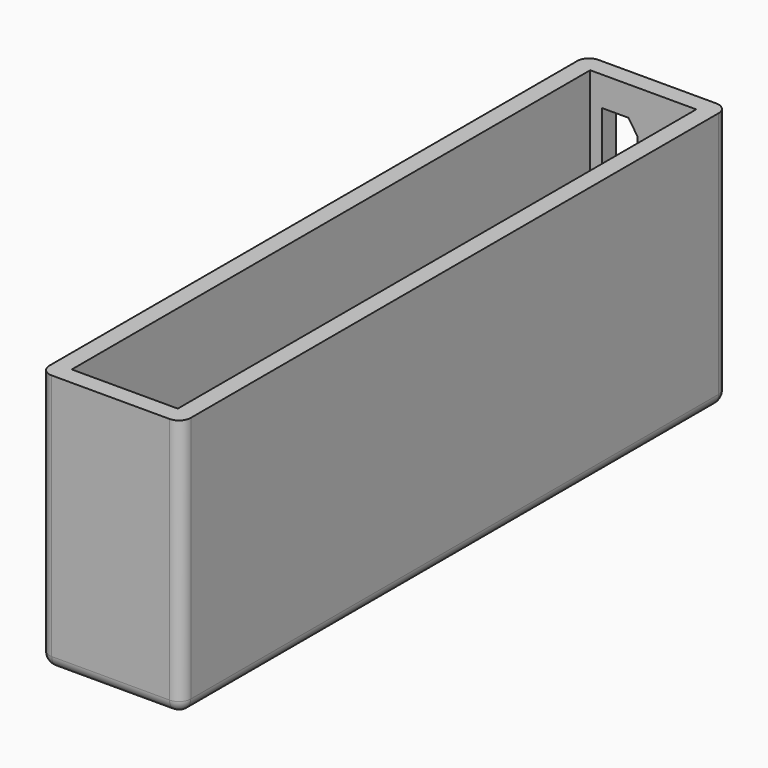
from build123d import *

# Parameters (mm, degrees)
F0_W          = 24
F0_H          = 116
F1_DEPTH      = 44
F2_T          = -3
F3_W          = 8.5
F3_H          = 16.5
F3_W_2        = 10.6
F3_H_2        = 12.5
F4_DEPTH      = 25
F5_W          = 6
F5_H          = 15.5
F6_DEPTH      = 25
F7_SIZE2      = 2.25
F7_SIZE       = 1.5
F9_DEPTH      = 7
F10_R         = 2.4
F11_DEPTH     = 1.6
F12_R         = 2
F13_T1_DEPTH  = 47
F13_S5_W      = 2
F13_S5_H      = 2
F13_T6_DEPTH  = 2
F13_S11_W     = 2
F13_S11_H     = 2
F13_T12_DEPTH = 2
F13_S17_W     = 2
F13_S17_H     = 2
F13_T18_DEPTH = 2
F13_S23_W     = 2
F13_S23_H     = 2
F13_T24_DEPTH = 2


# Not quite as in the source:
# - a fillet or chamfer that OpenCascade refuses, or shapes differently, is made with other operations: its cross-section is extruded or revolved along the edge and cut away or added


with BuildPart() as f1:
    # F0 (on Top) → F1 (new body)
    with BuildSketch(Plane.XY):
        Rectangle(F0_W, F0_H)
    extrude(amount=F1_DEPTH)

    # F2
    f2_openings = [f1.faces().sort_by_distance(p)[0] for p in [
        (0, 0, 44),
    ]]
    offset(amount=F2_T, openings=f2_openings)

    # F3 (on face) → F4 (cut)
    with BuildSketch(Plane(origin=(0, 0, 0), x_dir=(1, 0, 0), z_dir=(0, 0, -1))):
        with Locations((-4.75, 9.75)):
            Rectangle(F3_W, F3_H)
        with Locations((-3.7, -11.75)):
            Rectangle(F3_W_2, F3_H_2)
    extrude(amount=-F4_DEPTH, mode=Mode.SUBTRACT)

    # F5 (on face) → F6 (cut)
    with BuildSketch(Plane(origin=(0, 58, 0), x_dir=(-1, 0, 0), z_dir=(0, 1, 0))):
        with Locations((4, 31.25)):
            Rectangle(F5_W, F5_H)
    extrude(amount=-F6_DEPTH, mode=Mode.SUBTRACT)

    # F7
    f7_edges = [f1.edges().sort_by_distance(p)[0] for p in [
        (-1, 56.5, 23.5),
        (-1, 56.5, 39),
    ]]
    chamfer(f7_edges, length=F7_SIZE, length2=F7_SIZE2)

    # F8 (on face) → F9 (join)
    with BuildSketch(Plane.XY.offset(3)):
        Polygon((4.6, 21), (-9, 21), (-9, 18), (1.6, 18), (1.6, 5.5), (-9, 5.5), (-9, 2.5), (4.6, 2.5), align=None)
        Polygon((-9, -18), (-9, -21), (2.5, -21), (2.5, 1.5), (-9, 1.5), (-9, -1.5), (-0.5, -1.5), (-0.5, -18), align=None)
    extrude(amount=F9_DEPTH)

    # F10 (on face) → F11 (join)
    with BuildSketch(Plane(origin=(-12, 0, 0), x_dir=(0, -1, 0), z_dir=(-1, 0, 0))):
        with Locations((-52, 6)):
            Circle(F10_R)
        with Locations((-52, 14)):
            Circle(F10_R)
        with Locations((-52, 22)):
            Circle(F10_R)
        with Locations((-52, 30)):
            Circle(F10_R)
        with Locations((-52, 38)):
            Circle(F10_R)
        with Locations((-44, 6)):
            Circle(F10_R)
        with Locations((-44, 14)):
            Circle(F10_R)
        with Locations((-44, 22)):
            Circle(F10_R)
        with Locations((-44, 30)):
            Circle(F10_R)
        with Locations((-44, 38)):
            Circle(F10_R)
        with Locations((-36, 6)):
            Circle(F10_R)
        with Locations((-36, 14)):
            Circle(F10_R)
        with Locations((-36, 22)):
            Circle(F10_R)
        with Locations((-36, 30)):
            Circle(F10_R)
        with Locations((-36, 38)):
            Circle(F10_R)
        with Locations((-28, 6)):
            Circle(F10_R)
        with Locations((-28, 14)):
            Circle(F10_R)
        with Locations((-28, 22)):
            Circle(F10_R)
        with Locations((-28, 30)):
            Circle(F10_R)
        with Locations((-28, 38)):
            Circle(F10_R)
        with Locations((-20, 6)):
            Circle(F10_R)
        with Locations((-20, 14)):
            Circle(F10_R)
        with Locations((-20, 22)):
            Circle(F10_R)
        with Locations((-20, 30)):
            Circle(F10_R)
        with Locations((-20, 38)):
            Circle(F10_R)
        with Locations((-12, 6)):
            Circle(F10_R)
        with Locations((-12, 14)):
            Circle(F10_R)
        with Locations((-12, 22)):
            Circle(F10_R)
        with Locations((-12, 30)):
            Circle(F10_R)
        with Locations((-12, 38)):
            Circle(F10_R)
        with Locations((-4, 6)):
            Circle(F10_R)
        with Locations((-4, 14)):
            Circle(F10_R)
        with Locations((-4, 22)):
            Circle(F10_R)
        with Locations((-4, 30)):
            Circle(F10_R)
        with Locations((-4, 38)):
            Circle(F10_R)
        with Locations((4, 6)):
            Circle(F10_R)
        with Locations((4, 14)):
            Circle(F10_R)
        with Locations((4, 22)):
            Circle(F10_R)
        with Locations((4, 30)):
            Circle(F10_R)
        with Locations((4, 38)):
            Circle(F10_R)
        with Locations((12, 6)):
            Circle(F10_R)
        with Locations((12, 14)):
            Circle(F10_R)
        with Locations((12, 22)):
            Circle(F10_R)
        with Locations((12, 30)):
            Circle(F10_R)
        with Locations((12, 38)):
            Circle(F10_R)
        with Locations((20, 6)):
            Circle(F10_R)
        with Locations((20, 14)):
            Circle(F10_R)
        with Locations((20, 22)):
            Circle(F10_R)
        with Locations((20, 30)):
            Circle(F10_R)
        with Locations((20, 38)):
            Circle(F10_R)
        with Locations((28, 6)):
            Circle(F10_R)
        with Locations((28, 14)):
            Circle(F10_R)
        with Locations((28, 22)):
            Circle(F10_R)
        with Locations((28, 30)):
            Circle(F10_R)
        with Locations((28, 38)):
            Circle(F10_R)
        with Locations((36, 6)):
            Circle(F10_R)
        with Locations((36, 14)):
            Circle(F10_R)
        with Locations((36, 22)):
            Circle(F10_R)
        with Locations((36, 30)):
            Circle(F10_R)
        with Locations((36, 38)):
            Circle(F10_R)
        with Locations((44, 6)):
            Circle(F10_R)
        with Locations((44, 14)):
            Circle(F10_R)
        with Locations((44, 22)):
            Circle(F10_R)
        with Locations((44, 30)):
            Circle(F10_R)
        with Locations((44, 38)):
            Circle(F10_R)
        with Locations((52, 6)):
            Circle(F10_R)
        with Locations((52, 14)):
            Circle(F10_R)
        with Locations((52, 22)):
            Circle(F10_R)
        with Locations((52, 30)):
            Circle(F10_R)
        with Locations((52, 38)):
            Circle(F10_R)
    extrude(amount=F11_DEPTH)

    # F12
    f12_edges = [f1.edges().sort_by_distance(p)[0] for p in [
        (12, 0, 0),
        (0, -58, 0),
        (-12, 0, 0),
        (0, 58, 0),
    ]]
    fillet(f12_edges, radius=F12_R)

    # F13: fillet of radius 2 on 4 edges, made by hand

    # F13_s2 → F13_t1 (cut)
    with BuildSketch(Plane.XY.offset(2)):
        with BuildLine():
            ThreePointArc((-12, -56), (-11.4142135624, -57.4142135624), (-10, -58))
            Line((-10, -58), (-12, -58))
            Line((-12, -58), (-12, -56))
        make_face()
        with BuildLine():
            ThreePointArc((12, -56), (11.4142135624, -57.4142135624), (10, -58))
            Line((10, -58), (12, -58))
            Line((12, -58), (12, -56))
        make_face()
        with BuildLine():
            ThreePointArc((10, 58), (11.4142135624, 57.4142135624), (12, 56))
            Line((12, 56), (12, 58))
            Line((12, 58), (10, 58))
        make_face()
        with BuildLine():
            ThreePointArc((-10, 58), (-11.4142135624, 57.4142135624), (-12, 56))
            Line((-12, 56), (-12, 58))
            Line((-12, 58), (-10, 58))
        make_face()
    extrude(amount=F13_T1_DEPTH, mode=Mode.SUBTRACT)


with BuildPart() as f13_tool4:
    # F13_s5 → F13_t6 (new body)
    with BuildSketch(Plane.XZ.offset(-56)):
        with Locations((-11, 1)):
            Rectangle(F13_S5_W, F13_S5_H)
    extrude(amount=-F13_T6_DEPTH)

    # F13_s7 → F13_t8 (revolve, cut)
    with BuildSketch(Plane(origin=(-10, 56, 2), x_dir=(0.7071067812, 0, 0.7071067812), z_dir=(-0.7071067812, 0, 0.7071067812))):
        with BuildLine():
            ThreePointArc((0, -2), (2, 0), (0, 2))
            Line((0, 2), (0, -2))
        make_face()
    revolve(axis=Axis((-10, 56, 2), (0, 1, 0)), mode=Mode.SUBTRACT)


with BuildPart() as f1_1:
    add(f1.part)

    # F13_t3: cut F13_tool4
    add(f13_tool4.part, mode=Mode.SUBTRACT)


with BuildPart() as f13_tool10:
    # F13_s11 → F13_t12 (new body)
    with BuildSketch(Plane.XZ.offset(-56)):
        with Locations((11, 1)):
            Rectangle(F13_S11_W, F13_S11_H)
    extrude(amount=-F13_T12_DEPTH)

    # F13_s13 → F13_t14 (revolve, cut)
    with BuildSketch(Plane(origin=(10, 56, 2), x_dir=(-0.7071067812, 0, 0.7071067812), z_dir=(-0.7071067812, 0, -0.7071067812))):
        with BuildLine():
            ThreePointArc((0, -2), (2, 0), (0, 2))
            Line((0, 2), (0, -2))
        make_face()
    revolve(axis=Axis((10, 56, 2), (0, 1, 0)), mode=Mode.SUBTRACT)


with BuildPart() as f1_2:
    add(f1_1.part)

    # F13_t9: cut F13_tool10
    add(f13_tool10.part, mode=Mode.SUBTRACT)


with BuildPart() as f13_tool16:
    # F13_s17 → F13_t18 (new body)
    with BuildSketch(Plane.YZ.offset(10)):
        with Locations((-57, 1)):
            Rectangle(F13_S17_W, F13_S17_H)
    extrude(amount=F13_T18_DEPTH)

    # F13_s19 → F13_t20 (revolve, cut)
    with BuildSketch(Plane(origin=(10, -56, 2), x_dir=(0, 0.7071067812, 0.7071067812), z_dir=(0, 0.7071067812, -0.7071067812))):
        with BuildLine():
            ThreePointArc((0, -2), (2, 0), (0, 2))
            Line((0, 2), (0, -2))
        make_face()
    revolve(axis=Axis((10, -56, 2), (1, 0, 0)), mode=Mode.SUBTRACT)


with BuildPart() as f1_3:
    add(f1_2.part)

    # F13_t15: cut F13_tool16
    add(f13_tool16.part, mode=Mode.SUBTRACT)


with BuildPart() as f13_tool22:
    # F13_s23 → F13_t24 (new body)
    with BuildSketch(Plane.YZ.offset(-10)):
        with Locations((-57, 1)):
            Rectangle(F13_S23_W, F13_S23_H)
    extrude(amount=-F13_T24_DEPTH)

    # F13_s25 → F13_t26 (revolve, cut)
    with BuildSketch(Plane(origin=(-10, -56, 2), x_dir=(0, 0.7071067812, 0.7071067812), z_dir=(0, -0.7071067812, 0.7071067812))):
        with BuildLine():
            ThreePointArc((0, -2), (2, 0), (0, 2))
            Line((0, 2), (0, -2))
        make_face()
    revolve(axis=Axis((-10, -56, 2), (-1, 0, 0)), mode=Mode.SUBTRACT)


with BuildPart() as f1_4:
    add(f1_3.part)

    # F13_t21: cut F13_tool22
    add(f13_tool22.part, mode=Mode.SUBTRACT)


solid = f1_4.part
